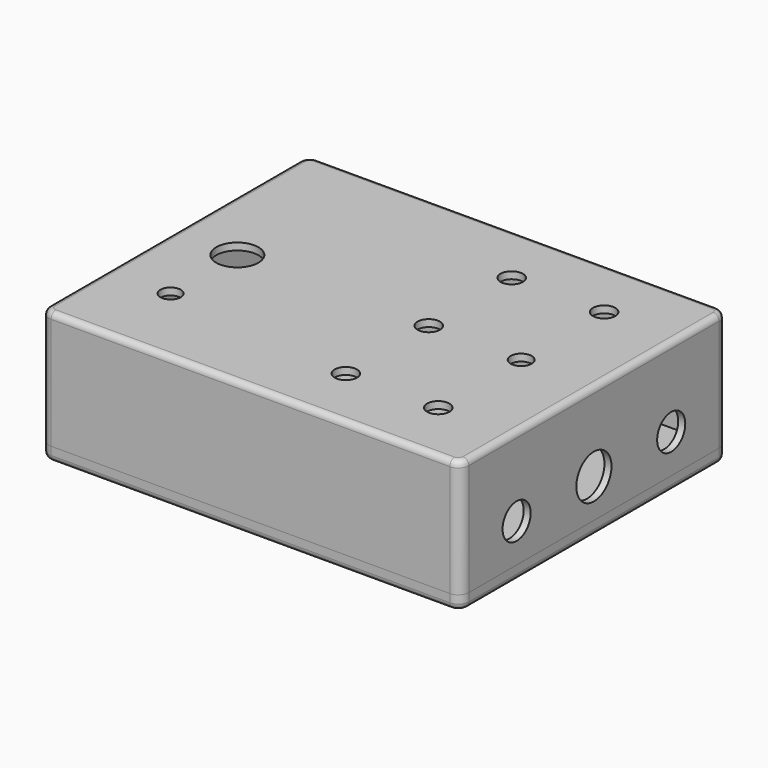
from build123d import *

# Parameters (mm, degrees)
F1_DEPTH        = 33.5
F3_DEPTH        = 31.5
F5_DEPTH        = 2.5
F6_R            = 2
F7_DEPTH        = 25
F8_DEPTH        = 4
F9_DEPTH        = 4.001
F10_SIZE        = 1.5
F11_T1_DEPTH    = 89
F11_T3_DEPTH    = 113.5
F11_T6_ANGLE    = 90
F11_T8_ANGLE    = 90
F11_T10_ANGLE   = 90
F11_T12_ANGLE   = 90
F11_2_T1_DEPTH  = 89
F11_2_T3_DEPTH  = 113.5
F11_2_T8_ANGLE  = 90
F11_2_T10_ANGLE = 90
F11_2_T12_ANGLE = 90
F11_2_T14_ANGLE = 90
F12_R           = 3.175
F12_R_2         = 3
F12_R_3         = 6
F12_R_4         = 2.9
F13_DEPTH       = 2
F14_R           = 5
F14_R_2         = 6.25
F15_DEPTH       = 25


# Not quite as in the source:
# - a fillet or chamfer that OpenCascade refuses, or shapes differently, is made with other operations: its cross-section is extruded or revolved along the edge and cut away or added


with BuildPart() as f1:
    # F0 (on Top) → F1 (new body)
    with BuildSketch(Plane.XY):
        with BuildLine():
            ThreePointArc((0, 3), (0.8786796564, 0.8786796564), (3, 0))
            Line((3, 0), (116.5, 0))
            ThreePointArc((116.5, 0), (118.6213203436, 0.8786796564), (119.5, 3))
            Line((119.5, 3), (119.5, 92))
            ThreePointArc((119.5, 92), (118.6213203436, 94.1213203436), (116.5, 95))
            Line((116.5, 95), (3, 95))
            ThreePointArc((3, 95), (0.8786796564, 94.1213203436), (0, 92))
            Line((0, 92), (0, 3))
        make_face()
    extrude(amount=F1_DEPTH)

    # F2 (on face) → F3 (cut)
    with BuildSketch(Plane(origin=(0, 0, 0), x_dir=(1, 0, 0), z_dir=(0, 0, -1))):
        with BuildLine():
            Line((111.5, -2), (8, -2))
            Line((8, -2), (8, -6))
            ThreePointArc((8, -6), (7.4142135624, -7.4142135624), (6, -8))
            Line((6, -8), (2, -8))
            Line((2, -8), (2, -87))
            Line((2, -87), (6, -87))
            ThreePointArc((6, -87), (7.4142135624, -87.5857864376), (8, -89))
            Line((8, -89), (8, -93))
            Line((8, -93), (111.5, -93))
            Line((111.5, -93), (111.5, -89))
            ThreePointArc((111.5, -89), (112.0857864376, -87.5857864376), (113.5, -87))
            Line((113.5, -87), (117.5, -87))
            Line((117.5, -87), (117.5, -8))
            Line((117.5, -8), (113.5, -8))
            ThreePointArc((113.5, -8), (112.0857864376, -7.4142135624), (111.5, -6))
            Line((111.5, -6), (111.5, -2))
        make_face()
    extrude(amount=-F3_DEPTH, mode=Mode.SUBTRACT)

    # F4 (on face) → F5 (cut)
    with BuildSketch(Plane(origin=(0, 0, 0), x_dir=(1, 0, 0), z_dir=(0, 0, -1))):
        with BuildLine():
            Line((8, -6), (8, -2))
            Line((8, -2), (4, -2))
            ThreePointArc((4, -2), (2.5857864376, -2.5857864376), (2, -4))
            Line((2, -4), (2, -8))
            Line((2, -8), (6, -8))
            ThreePointArc((6, -8), (7.4142135624, -7.4142135624), (8, -6))
        make_face()
        with BuildLine():
            Line((115.5, -2), (111.5, -2))
            Line((111.5, -2), (111.5, -6))
            ThreePointArc((111.5, -6), (112.0857864376, -7.4142135624), (113.5, -8))
            Line((113.5, -8), (117.5, -8))
            Line((117.5, -8), (117.5, -4))
            ThreePointArc((117.5, -4), (116.9142135624, -2.5857864376), (115.5, -2))
        make_face()
        with BuildLine():
            Line((117.5, -91), (117.5, -87))
            Line((117.5, -87), (113.5, -87))
            ThreePointArc((113.5, -87), (112.0857864376, -87.5857864376), (111.5, -89))
            Line((111.5, -89), (111.5, -93))
            Line((111.5, -93), (115.5, -93))
            ThreePointArc((115.5, -93), (116.9142135624, -92.4142135624), (117.5, -91))
        make_face()
        with BuildLine():
            Line((6, -87), (2, -87))
            Line((2, -87), (2, -91))
            ThreePointArc((2, -91), (2.5857864376, -92.4142135624), (4, -93))
            Line((4, -93), (8, -93))
            Line((8, -93), (8, -89))
            ThreePointArc((8, -89), (7.4142135624, -87.5857864376), (6, -87))
        make_face()
    extrude(amount=-F5_DEPTH, mode=Mode.SUBTRACT)

    # F6 (on face) → F7 (cut)
    with BuildSketch(Plane(origin=(0, 0, 0), x_dir=(1, 0, 0), z_dir=(0, 0, -1))):
        with Locations((5, -5)):
            Circle(F6_R)
        with Locations((114.5, -5)):
            Circle(F6_R)
        with Locations((114.5, -90)):
            Circle(F6_R)
        with Locations((5, -90)):
            Circle(F6_R)
    extrude(amount=-F7_DEPTH, mode=Mode.SUBTRACT)

    # F11: fillet of radius 1.7 on 8 edges, made by hand

    # F11_s2 → F11_t1 (cut)
    with BuildSketch(Plane.XZ.offset(-92)):
        with BuildLine():
            ThreePointArc((0, 31.8), (0.497918472, 33.002081528), (1.7, 33.5))
            Line((1.7, 33.5), (0, 33.5))
            Line((0, 33.5), (0, 31.8))
        make_face()
        with BuildLine():
            ThreePointArc((117.8, 33.5), (119.002081528, 33.002081528), (119.5, 31.8))
            Line((119.5, 31.8), (119.5, 33.5))
            Line((119.5, 33.5), (117.8, 33.5))
        make_face()
    extrude(amount=F11_T1_DEPTH, mode=Mode.SUBTRACT)

    # F11_s4 → F11_t3 (cut)
    with BuildSketch(Plane.YZ.offset(3)):
        with BuildLine():
            ThreePointArc((1.7, 33.5), (0.497918472, 33.002081528), (0, 31.8))
            Line((0, 31.8), (0, 33.5))
            Line((0, 33.5), (1.7, 33.5))
        make_face()
        with BuildLine():
            ThreePointArc((93.3, 33.5), (94.502081528, 33.002081528), (95, 31.8))
            Line((95, 31.8), (95, 33.5))
            Line((95, 33.5), (93.3, 33.5))
        make_face()
    extrude(amount=F11_T3_DEPTH, mode=Mode.SUBTRACT)

    # F11_s5 → F11_t6 (revolve, cut)
    with BuildSketch(Plane.XZ.offset(-3)):
        with BuildLine():
            ThreePointArc((0, 31.8), (0.497918472, 33.002081528), (1.7, 33.5))
            Line((1.7, 33.5), (0, 33.5))
            Line((0, 33.5), (0, 31.8))
        make_face()
    revolve(axis=Axis((3, 3, 33.5), (0, 0, 1)), revolution_arc=F11_T6_ANGLE, mode=Mode.SUBTRACT)

    # F11_s7 → F11_t8 (revolve, cut)
    with BuildSketch(Plane.YZ.offset(116.5)):
        with BuildLine():
            ThreePointArc((1.7, 33.5), (0.497918472, 33.002081528), (0, 31.8))
            Line((0, 31.8), (0, 33.5))
            Line((0, 33.5), (1.7, 33.5))
        make_face()
    revolve(axis=Axis((116.5, 3, 33.5), (0, 0, 1)), revolution_arc=F11_T8_ANGLE, mode=Mode.SUBTRACT)

    # F11_s9 → F11_t10 (revolve, cut)
    with BuildSketch(Plane.XZ.offset(-92)):
        with BuildLine():
            ThreePointArc((117.8, 33.5), (119.002081528, 33.002081528), (119.5, 31.8))
            Line((119.5, 31.8), (119.5, 33.5))
            Line((119.5, 33.5), (117.8, 33.5))
        make_face()
    revolve(axis=Axis((116.5, 92, 33.5), (0, 0, 1)), revolution_arc=F11_T10_ANGLE, mode=Mode.SUBTRACT)

    # F11_s11 → F11_t12 (revolve, cut)
    with BuildSketch(Plane.YZ.offset(3)):
        with BuildLine():
            ThreePointArc((95, 31.8), (94.502081528, 33.002081528), (93.3, 33.5))
            Line((93.3, 33.5), (95, 33.5))
            Line((95, 33.5), (95, 31.8))
        make_face()
    revolve(axis=Axis((3, 92, 33.5), (0, 0, 1)), revolution_arc=F11_T12_ANGLE, mode=Mode.SUBTRACT)

    # F12 (on face) → F13 (cut, through all)
    with BuildSketch(Plane.XY.offset(33.5)):
        with Locations((72.5, 77)):
            Circle(F12_R)
        with Locations((72.5, 18)):
            Circle(F12_R)
        with Locations((72.5, 47.5)):
            Circle(F12_R)
        with Locations((98.8, 77)):
            Circle(F12_R)
        with Locations((98.8, 18)):
            Circle(F12_R)
        with Locations((98.8, 47.5)):
            Circle(F12_R_2)
        with Locations((18, 47.5)):
            Circle(F12_R_3)
        with Locations((18, 23.75)):
            Circle(F12_R_4)
    extrude(amount=-F13_DEPTH, mode=Mode.SUBTRACT)

    # F14 (on face) → F15 (cut)
    with BuildSketch(Plane.YZ.offset(119.5)):
        with Locations((20, 11)):
            Circle(F14_R)
        with Locations((75, 11)):
            Circle(F14_R)
        with Locations((47.5, 11)):
            Circle(F14_R_2)
    extrude(amount=-F15_DEPTH, mode=Mode.SUBTRACT)


with BuildPart() as f8:
    # F0 (on Top) → F8 (new body)
    with BuildSketch(Plane.XY):
        with BuildLine():
            ThreePointArc((0, 3), (0.8786796564, 0.8786796564), (3, 0))
            Line((3, 0), (116.5, 0))
            ThreePointArc((116.5, 0), (118.6213203436, 0.8786796564), (119.5, 3))
            Line((119.5, 3), (119.5, 92))
            ThreePointArc((119.5, 92), (118.6213203436, 94.1213203436), (116.5, 95))
            Line((116.5, 95), (3, 95))
            ThreePointArc((3, 95), (0.8786796564, 94.1213203436), (0, 92))
            Line((0, 92), (0, 3))
        make_face()
    extrude(amount=-F8_DEPTH)

    # F6 (on face) → F9 (cut, through all)
    with BuildSketch(Plane(origin=(0, 0, 0), x_dir=(1, 0, 0), z_dir=(0, 0, -1))):
        with Locations((5, -5)):
            Circle(F6_R)
        with Locations((114.5, -5)):
            Circle(F6_R)
        with Locations((114.5, -90)):
            Circle(F6_R)
        with Locations((5, -90)):
            Circle(F6_R)
    extrude(amount=F9_DEPTH, mode=Mode.SUBTRACT)

    # F10
    f10_edges = [f8.edges().sort_by_distance(p)[0] for p in [
        (3, 5, -4),
        (112.5, 5, -4),
        (112.5, 90, -4),
        (3, 90, -4),
    ]]
    chamfer(f10_edges, length=F10_SIZE)

    # F11#2: fillet of radius 1.7 on 12 edges, made by hand

    # F11_2_s2 → F11_2_t1 (cut)
    with BuildSketch(Plane.XZ.offset(-92)):
        with BuildLine():
            ThreePointArc((1.7, -4), (0.497918472, -3.502081528), (0, -2.3))
            Line((0, -2.3), (0, -4))
            Line((0, -4), (1.7, -4))
        make_face()
        with BuildLine():
            ThreePointArc((117.8, -4), (119.002081528, -3.502081528), (119.5, -2.3))
            Line((119.5, -2.3), (119.5, -4))
            Line((119.5, -4), (117.8, -4))
        make_face()
    extrude(amount=F11_2_T1_DEPTH, mode=Mode.SUBTRACT)

    # F11_2_s4 → F11_2_t3 (cut)
    with BuildSketch(Plane.YZ.offset(3)):
        with BuildLine():
            ThreePointArc((93.3, -4), (94.502081528, -3.502081528), (95, -2.3))
            Line((95, -2.3), (95, -4))
            Line((95, -4), (93.3, -4))
        make_face()
        with BuildLine():
            ThreePointArc((1.7, -4), (0.497918472, -3.502081528), (0, -2.3))
            Line((0, -2.3), (0, -4))
            Line((0, -4), (1.7, -4))
        make_face()
    extrude(amount=F11_2_T3_DEPTH, mode=Mode.SUBTRACT)

    # F11_2_s5 → F11_2_t6 (revolve, cut)
    with BuildSketch(Plane.XZ.offset(-5)):
        with BuildLine():
            ThreePointArc((9.204163056, -4), (8.553601221, -3.8705952053), (8.002081528, -3.502081528))
            Line((8.002081528, -3.502081528), (8.5, -4))
            Line((8.5, -4), (9.204163056, -4))
        make_face()
    revolve(axis=Axis((5, 5, -4), (0, 0, 1)), mode=Mode.SUBTRACT)

    # F11_2_s7 → F11_2_t8 (revolve, cut)
    with BuildSketch(Plane.YZ.offset(3)):
        with BuildLine():
            ThreePointArc((93.3, -4), (94.502081528, -3.502081528), (95, -2.3))
            Line((95, -2.3), (95, -4))
            Line((95, -4), (93.3, -4))
        make_face()
    revolve(axis=Axis((3, 92, -4), (0, 0, 1)), revolution_arc=F11_2_T8_ANGLE, mode=Mode.SUBTRACT)

    # F11_2_s9 → F11_2_t10 (revolve, cut)
    with BuildSketch(Plane.XZ.offset(-3)):
        with BuildLine():
            ThreePointArc((1.7, -4), (0.497918472, -3.502081528), (0, -2.3))
            Line((0, -2.3), (0, -4))
            Line((0, -4), (1.7, -4))
        make_face()
    revolve(axis=Axis((3, 3, -4), (0, 0, 1)), revolution_arc=F11_2_T10_ANGLE, mode=Mode.SUBTRACT)

    # F11_2_s11 → F11_2_t12 (revolve, cut)
    with BuildSketch(Plane.XZ.offset(-92)):
        with BuildLine():
            ThreePointArc((117.8, -4), (119.002081528, -3.502081528), (119.5, -2.3))
            Line((119.5, -2.3), (119.5, -4))
            Line((119.5, -4), (117.8, -4))
        make_face()
    revolve(axis=Axis((116.5, 92, -4), (0, 0, 1)), revolution_arc=F11_2_T12_ANGLE, mode=Mode.SUBTRACT)

    # F11_2_s13 → F11_2_t14 (revolve, cut)
    with BuildSketch(Plane.YZ.offset(116.5)):
        with BuildLine():
            ThreePointArc((1.7, -4), (0.497918472, -3.502081528), (0, -2.3))
            Line((0, -2.3), (0, -4))
            Line((0, -4), (1.7, -4))
        make_face()
    revolve(axis=Axis((116.5, 3, -4), (0, 0, 1)), revolution_arc=F11_2_T14_ANGLE, mode=Mode.SUBTRACT)

    # F11_2_s15 → F11_2_t16 (revolve, cut)
    with BuildSketch(Plane.XZ.offset(-5)):
        with BuildLine():
            ThreePointArc((118.704163056, -4), (118.053601221, -3.8705952053), (117.502081528, -3.502081528))
            Line((117.502081528, -3.502081528), (118, -4))
            Line((118, -4), (118.704163056, -4))
        make_face()
    revolve(axis=Axis((114.5, 5, -4), (0, 0, 1)), mode=Mode.SUBTRACT)

    # F11_2_s17 → F11_2_t18 (revolve, cut)
    with BuildSketch(Plane.XZ.offset(-90)):
        with BuildLine():
            ThreePointArc((118.704163056, -4), (118.053601221, -3.8705952053), (117.502081528, -3.502081528))
            Line((117.502081528, -3.502081528), (118, -4))
            Line((118, -4), (118.704163056, -4))
        make_face()
    revolve(axis=Axis((114.5, 90, -4), (0, 0, 1)), mode=Mode.SUBTRACT)

    # F11_2_s19 → F11_2_t20 (revolve, cut)
    with BuildSketch(Plane.XZ.offset(-90)):
        with BuildLine():
            ThreePointArc((9.204163056, -4), (8.553601221, -3.8705952053), (8.002081528, -3.502081528))
            Line((8.002081528, -3.502081528), (8.5, -4))
            Line((8.5, -4), (9.204163056, -4))
        make_face()
    revolve(axis=Axis((5, 90, -4), (0, 0, 1)), mode=Mode.SUBTRACT)


solid = Compound([f1.part, f8.part])
